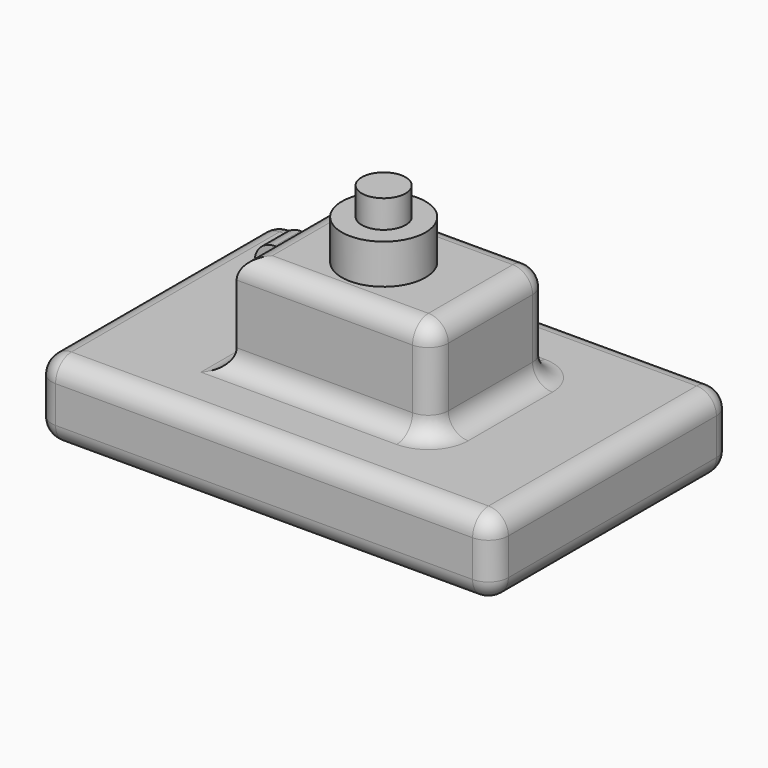
from build123d import *

# Parameters (mm, degrees)
F0_W        = 116.8206892908
F0_H        = 76.6635760665
F1_DEPTH    = 19.558
F2_R        = 5.08
F3_W        = 50.0696562231
F3_H        = 37.0959769934
F4_DEPTH    = 25.4
F5_F1_R     = 5.08
F5_F2_R     = 5.08
F6_W        = 18.107265234
F6_H        = 8.2995928824
F7_DEPTH    = 4.318
F8_T1_DEPTH = 33.4122171977
F9_R        = 10.7094586845
F10_DEPTH   = 10.16
F11_R       = 5.6111694278
F12_DEPTH   = 7.112


# Not quite as in the source:
# - a fillet or chamfer that OpenCascade refuses, or shapes differently, is made with other operations: its cross-section is extruded or revolved along the edge and cut away or added


with BuildPart() as f1:
    # F0 (on Top) → F1 (new body)
    with BuildSketch(Plane.XY):
        with Locations((-1.5465151519, 2.0281374454)):
            Rectangle(F0_W, F0_H)
    extrude(amount=F1_DEPTH)

    # F2
    f2_edges = [f1.edges().sort_by_distance(p)[0] for p in [
        (56.863829, 2.028137, 19.558),
        (-1.546515, 40.359925, 19.558),
        (-59.95686, 2.028137, 19.558),
        (-1.546515, -36.303651, 19.558),
        (-1.546515, -36.303651, 0),
        (56.863829, 2.028137, 0),
        (-1.546515, 40.359925, 0),
        (-59.95686, 2.028137, 0),
        (-59.95686, 40.359925, 9.779),
        (-59.95686, -36.303651, 9.779),
        (56.863829, 40.359925, 9.779),
        (56.863829, -36.303651, 9.779),
    ]]
    fillet(f2_edges, radius=F2_R)

    # F3 (on face) → F4 (join)
    with BuildSketch(Plane.XY.offset(19.558)):
        with Locations((0.8830688894, 1.7247768119)):
            Rectangle(F3_W, F3_H)
    extrude(amount=F4_DEPTH)

    # F5: fillet of radius 5.08 on 10 edges, made by hand

    # F5_f1
    f5_f1_edges = [f1.edges().sort_by_distance(p)[0] for p in [
        (0.8830688894, -16.8232116848, 44.958),
        (-24.1517592221, 1.7247768119, 44.958),
        (0.8830688894, 20.2727653086, 44.958),
        (25.9178970009, 1.7247768119, 44.958),
        (25.9178970009, -16.8232116848, 32.258),
        (25.9178970009, 20.2727653086, 32.258),
        (-24.1517592221, 20.2727653086, 32.258),
    ]]
    fillet(f5_f1_edges, radius=F5_F1_R)

    # F5_f2
    f5_f2_edges = [f1.edges().sort_by_distance(p)[0] for p in [
        (25.9178970009, 1.7247768119, 19.558),
        (-24.1517592221, -0.8152231881, 19.558),
        (0.8830688894, 20.2727653086, 19.558),
        (24.4299994493, 18.784867757, 19.558),
        (-22.6638616706, 18.784867757, 19.558),
        (24.4299994493, -15.3353141333, 19.558),
    ]]
    fillet(f5_f2_edges, radius=F5_F2_R)

    # F6 (on face) → F7 (join)
    with BuildSketch(Plane.XY.offset(19.558)):
        with Locations((-42.6498092711, 27.5764670223)):
            Rectangle(F6_W, F6_H)
    extrude(amount=F7_DEPTH)

    # F8: fillet of radius 5.08 on 2 edges, made by hand

    # F8_s2 → F8_t1 (cut)
    with BuildSketch(Plane.XZ.offset(-44.2825756211)):
        with BuildLine():
            ThreePointArc((-51.7034418881, 19.558), (-49.9926718469, 22.6481007256), (-46.680917025, 23.876))
            Line((-46.680917025, 23.876), (-51.7034418881, 23.876))
            Line((-51.7034418881, 23.876), (-51.7034418881, 19.558))
        make_face()
        with BuildLine():
            ThreePointArc((-33.5961766541, 19.558), (-35.3069466953, 22.6481007256), (-38.6187015172, 23.876))
            Line((-38.6187015172, 23.876), (-33.5961766541, 23.876))
            Line((-33.5961766541, 23.876), (-33.5961766541, 19.558))
        make_face()
    extrude(amount=F8_T1_DEPTH, mode=Mode.SUBTRACT)

    # F9 (on face) → F10 (join)
    with BuildSketch(Plane.XY.offset(44.958)):
        Circle(F9_R)
    extrude(amount=F10_DEPTH)

    # F11 (on face) → F12 (join)
    with BuildSketch(Plane.XY.offset(55.118)):
        Circle(F11_R)
    extrude(amount=F12_DEPTH)


solid = f1.part
